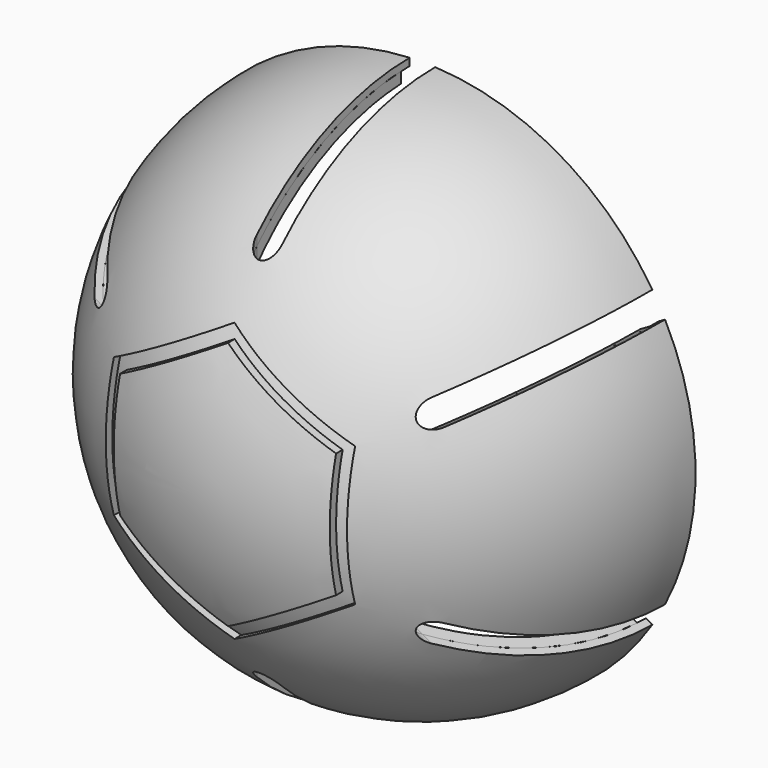
from build123d import *

# Parameters (mm, degrees)
F7_DEPTH  = 82.8
F14_DEPTH = 281.7029076382
F18_DEPTH = 206.7029076382
F19_DEPTH = 75.001
F20_DEPTH = 75.001


with BuildPart() as f1:
    # F0 (on Top) → F1 (revolve)
    with BuildSketch(Plane.XY):
        with BuildLine():
            Line((0, 0), (-75, 0))
            ThreePointArc((-75, 0), (-53.033008589, -53.033008589), (0, -75))
            Line((0, -75), (0, 0))
        make_face()
    revolve(axis=Axis((0, -37.5, 0), (0, -1, 0)))

    # F2 (on Top) → F3 (revolve, cut)
    with BuildSketch(Plane.XY):
        with BuildLine():
            Line((73, 0), (0, 0))
            Line((0, 0), (0, -73))
            ThreePointArc((0, -73), (51.6187950266, -51.6187950266), (73, 0))
        make_face()
    revolve(axis=Axis((0, -36.5, 0), (0, -1, 0)), mode=Mode.SUBTRACT)

    # F6 (on offset) → F7 (cut)
    with BuildSketch(Plane.XZ.offset(88)):
        Polygon((33.1254743015, 19.125001505), (0, 38.25000301), (-33.1254743015, 19.125001505), (-33.1254743015, -19.125001505), (0, -38.25000301), (33.1254743015, -19.125001505), align=None)
        Polygon((-29.6613721186, 17.1250011772), (0, 34.2500023544), (29.6613721186, 17.1250011772), (29.6613721186, -17.1250011772), (0, -34.2500023544), (-29.6613721186, -17.1250011772), align=None, mode=Mode.SUBTRACT)
    extrude(amount=-F7_DEPTH, mode=Mode.SUBTRACT)


with BuildPart() as f10:
    # F9 (on Top) → F10 (revolve)
    with BuildSketch(Plane.XY):
        with BuildLine():
            ThreePointArc((-0.003513299, -69.9999999118), (-48.4264685128, -50.5457925784), (-69.9356847396, -3))
            Line((-69.9356847396, -3), (-72.9383301152, -3))
            ThreePointArc((-72.9383301152, -3), (-50.548275215, -52.6675599662), (-0.003513299, -72.9999999155))
            Line((-0.003513299, -72.9999999155), (-0.003513299, -69.9999999118))
        make_face()
    revolve(axis=Axis((-0.003513299, -71.4999999136, 0), (0, -1, 0)))


with BuildPart() as f14_tool:
    # F13 (on face) → F14 (new body, through all)
    with BuildSketch(Plane(origin=(155.2350556673, 0, 89.6250011772), x_dir=(0, -1, 0), z_dir=(-0.8660254038, 0, -0.5))):
        with BuildLine():
            ThreePointArc((52.5, -3.4999984143), (56, 1.5857e-06), (52.5, 3.5000015857))
            Line((52.5, 3.5000015857), (0, 3.5000015857))
            Line((0, 3.5000015857), (0, -3.4999984143))
            Line((0, -3.4999984143), (52.5, -3.4999984143))
        make_face()
    extrude(amount=F14_DEPTH)


with BuildPart() as f1_1:
    add(f1.part)

    # F14: cut by f14_tool
    add(f14_tool.part, mode=Mode.SUBTRACT)


with BuildPart() as f10_1:
    add(f10.part)

    # F14: cut by f14_tool
    add(f14_tool.part, mode=Mode.SUBTRACT)


with BuildPart() as f18_tool:
    # F17 (on face) → F18 (new body, through all)
    with BuildSketch(Plane(origin=(90.2831503835, 0, -52.1250011772), x_dir=(0, -1, 0), z_dir=(-0.8660254038, 0, 0.5))):
        with BuildLine():
            ThreePointArc((52.5, -3.5), (56, 0), (52.5, 3.5))
            Line((52.5, 3.5), (0, 3.5))
            Line((0, 3.5), (0, -3.5))
            Line((0, -3.5), (52.5, -3.5))
        make_face()
    extrude(amount=F18_DEPTH)


with BuildPart() as f1_2:
    add(f1_1.part)

    # F18: cut by f18_tool
    add(f18_tool.part, mode=Mode.SUBTRACT)


with BuildPart() as f10_2:
    add(f10_1.part)

    # F18: cut by f18_tool
    add(f18_tool.part, mode=Mode.SUBTRACT)


with BuildPart() as f19_tool:
    # F4 (on Top) → F19 (new body, through all)
    with BuildSketch(Plane.XY):
        with BuildLine():
            ThreePointArc((-3.5, -52.5), (0, -56), (3.5, -52.5))
            Line((3.5, -52.5), (3.5, 0))
            Line((3.5, 0), (-3.5, 0))
            Line((-3.5, 0), (-3.5, -52.5))
        make_face()
    extrude(amount=-F19_DEPTH)


with BuildPart() as f1_3:
    add(f1_2.part)

    # F19: cut by f19_tool
    add(f19_tool.part, mode=Mode.SUBTRACT)


with BuildPart() as f10_3:
    add(f10_2.part)

    # F19: cut by f19_tool
    add(f19_tool.part, mode=Mode.SUBTRACT)


with BuildPart() as f20_tool:
    # F4 (on Top) → F20 (new body, through all)
    with BuildSketch(Plane.XY):
        with BuildLine():
            ThreePointArc((-3.5, -52.5), (0, -56), (3.5, -52.5))
            Line((3.5, -52.5), (3.5, 0))
            Line((3.5, 0), (-3.5, 0))
            Line((-3.5, 0), (-3.5, -52.5))
        make_face()
    extrude(amount=F20_DEPTH)


with BuildPart() as f1_4:
    add(f1_3.part)

    # F20: cut by f20_tool
    add(f20_tool.part, mode=Mode.SUBTRACT)


with BuildPart() as f10_4:
    add(f10_3.part)

    # F20: cut by f20_tool
    add(f20_tool.part, mode=Mode.SUBTRACT)


solid = Compound([f1_4.part, f10_4.part])
